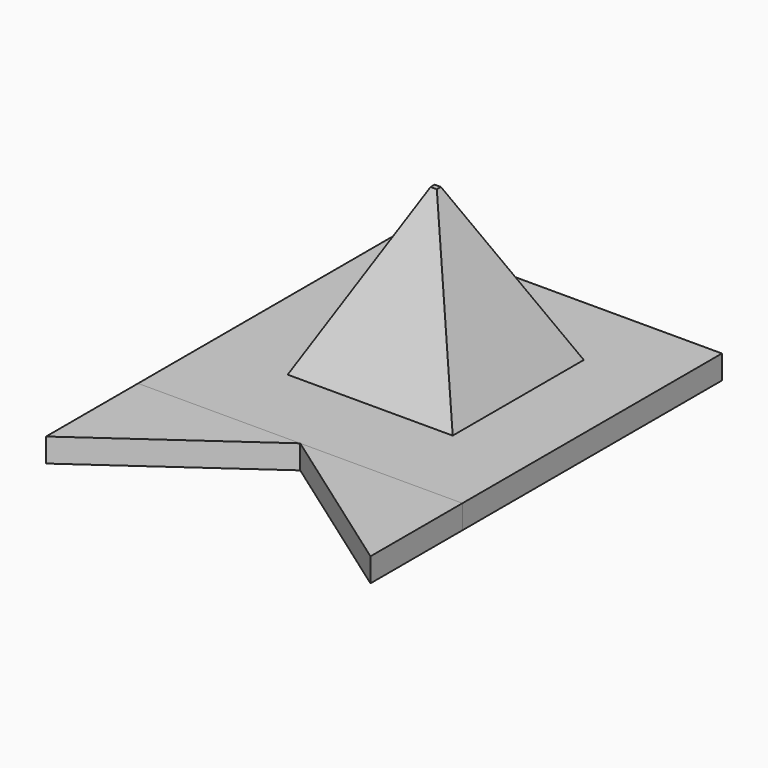
from build123d import *

# Parameters (mm, degrees)
F0_W     = 20.7871049643
F0_H     = 20.6407494843
F1_DEPTH = 20
F2_SIZE2 = 9.99999
F2_SIZE  = 19.99999
F3_W     = 40.8627185971
F3_H     = 40.862724185
F4_DEPTH = 3
F6_DEPTH = 3


# Not quite as in the source:
# - a fillet or chamfer is up to 0.001 mm smaller than in the source, because OpenCascade refuses the exact size


with BuildPart() as f1:
    # F0 (on Top) → F1 (new body)
    with BuildSketch(Plane.XY):
        with Locations((-28.3725745976, 20.8737719804)):
            Rectangle(F0_W, F0_H)
    extrude(amount=F1_DEPTH)

    # F2 (size 20 and 10 in the source; OpenCascade refuses exactly that, so slightly less here)
    f2_edges = [f1.edges().sort_by_distance(p)[0] for p in [
        (-17.979022, 20.873772, 20),
        (-38.766127, 20.873772, 20),
        (-28.372575, 10.553397, 20),
        (-28.372575, 31.194147, 20),
    ]]
    chamfer(f2_edges, length=F2_SIZE, length2=F2_SIZE2)

    # F3 (on face) → F4 (join)
    with BuildSketch(Plane(origin=(0, 0, 0), x_dir=(1, 0, 0), z_dir=(0, 0, -1))):
        with Locations((-28.6634135991, -20.3321799636)):
            Rectangle(F3_W, F3_H)
    extrude(amount=F4_DEPTH)


with BuildPart() as f6:
    # F5 (on face) → F6 (new body)
    with BuildSketch(Plane(origin=(0, 0, -3), x_dir=(1, 0, 0), z_dir=(0, 0, -1))):
        Polygon((-49.0947728977, 14.5796602592), (-49.0947728977, 0.0991821289), (-28.6634135991, 0.0991821289), align=None)
    extrude(amount=-F6_DEPTH)


with BuildPart() as f6b:
    # F5 (on face) → F6, piece 2 (new body)
    with BuildSketch(Plane(origin=(0, 0, -3), x_dir=(1, 0, 0), z_dir=(0, 0, -1))):
        Polygon((-8.2320543006, 14.5796602592), (-28.6634135991, 0.0991821289), (-8.2320543006, 0.0991821289), align=None)
    extrude(amount=-F6_DEPTH)


solid = Compound([f1.part, f6.part, f6b.part])
